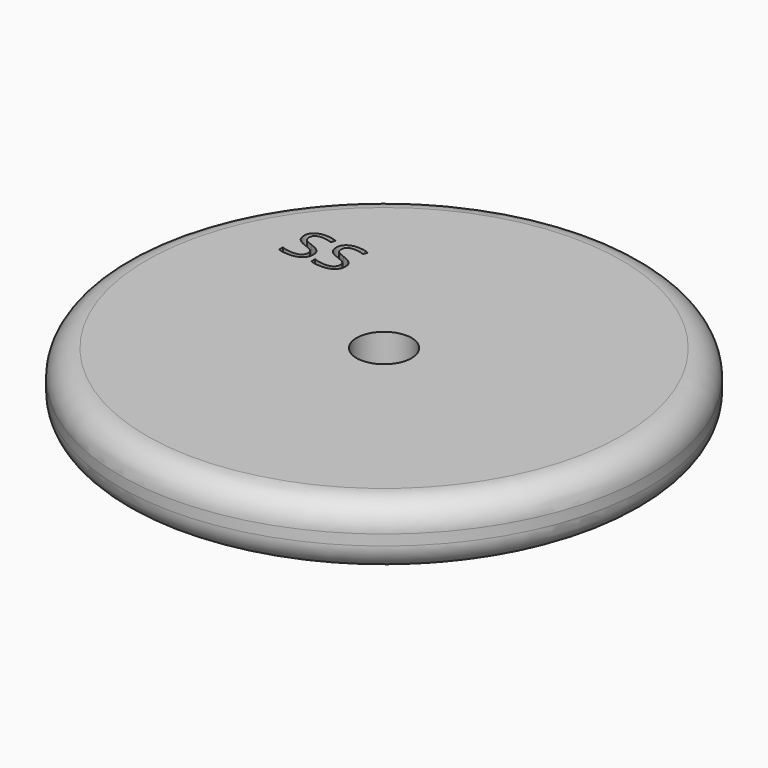
from build123d import *

# Parameters (mm, degrees)
F0_R         = 15.875
F1_DEPTH     = 3.81
F2_R         = 1.651
F3_DEPTH     = 3.811
F4_R         = 1.5875
F5_TEXT_SIZE = 3.5277777778
F6_DEPTH     = 3.175


# Not quite as in the source:
# - Text() gives the source's letters only with a copy of the font that has no kerning and outlines rounded to 1/6400 em; it was checked with that copy


with BuildPart() as f1:
    # F0 (on Top) → F1 (new body)
    with BuildSketch(Plane.XY):
        Circle(F0_R)
    extrude(amount=F1_DEPTH)

    # F2 (on face) → F3 (cut, through all)
    with BuildSketch(Plane.XY.offset(3.81)):
        Circle(F2_R)
    extrude(amount=-F3_DEPTH, mode=Mode.SUBTRACT)

    # F4
    f4_edges = [f1.edges().sort_by_distance(p)[0] for p in [
        (-15.875, 0, 3.81),
        (-15.875, 0, 0),
    ]]
    fillet(f4_edges, radius=F4_R)

    # F5 (on face) → F6 (cut)
    with BuildSketch(Plane.XY.offset(3.81)):
        with Locations((-10.2945903268, 4.6721558124)):
            Text('SS', F5_TEXT_SIZE, font='Open Sans', text_align=(TextAlign.LEFT, TextAlign.BOTTOM))
    extrude(amount=-F6_DEPTH, mode=Mode.SUBTRACT)


solid = f1.part
